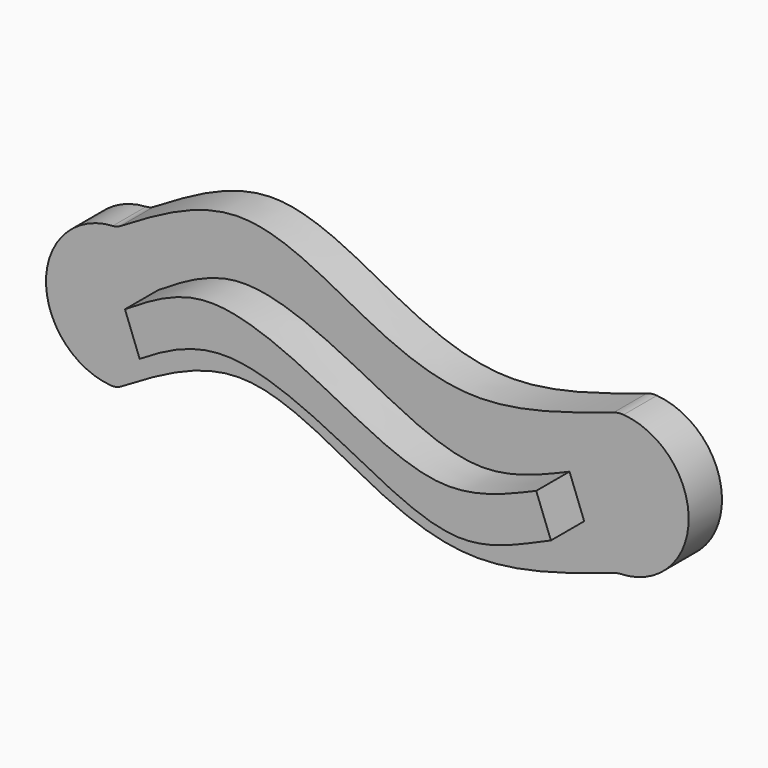
from build123d import *

# Parameters (mm, degrees)
F1_DEPTH = 12.7
F2_DEPTH = 25.4
F3_R     = 7.62
F4_R     = 5.08
F5_R     = 5.08
F6_R     = 5.08


# Not quite as in the source:
# - the program builds the solid bodies; features that only make, move or delete a surface that nothing else refers to are left out


with BuildPart() as f1:
    # F0 (on Front) → F1 (new body)
    with BuildSketch(Plane.XZ):
        with BuildLine():
            add(Edge.make_bspline(
                [(-76.5334740281, 20.7332828829), (-63.8515293548, 28.3869740492), (-38.487641079, 43.6943557355), (-0.1074870643, 19.2987869132), (33.6920782855, 6.372177087), (61.7287419774, 15.7705051868), (76.5334740281, 20.7332828829)],
                knots=[0, 0, 0, 0, 0.252598913, 0.5051978047, 0.7387201987, 1, 1, 1, 1], degree=3))
            Line((-76.5334740281, 20.7332828829), (-76.5334740281, -22.4467171171))
            add(Edge.make_bspline(
                [(-76.5334740281, -22.4467171171), (-63.8515293548, -14.7930259508), (-38.487641079, 0.5143557355), (-0.1074870643, -23.8812130868), (33.6920782855, -36.807822913), (61.7287419774, -27.4094948132), (76.5334740281, -22.4467171171)],
                knots=[0, 0, 0, 0, 0.252598913, 0.5051978047, 0.7387201987, 1, 1, 1, 1], degree=3))
            Line((76.5334740281, -22.4467171171), (76.5334740281, 20.7332828829))
        make_face()
        with BuildLine():
            Line((-59.3705394858, -3.9110629208), (-63.8515293548, 7.9721491784))
            add(Edge.make_bspline(
                [(-63.8515293548, 7.9721491784), (-55.8466582979, 13.0095149676), (-38.1452218943, 24.1488087208), (0.3419863459, 5.213337181), (32.9615149645, -12.272359942), (52.4893434663, -3.9416111996), (61.7287419774, 0)],
                knots=[0, 0, 0, 0, 0.228361581, 0.5049835251, 0.7657878611, 1, 1, 1, 1], degree=3))
            Line((61.7287419774, 0), (66.2097318464, -11.8832120992))
            add(Edge.make_bspline(
                [(-59.3705394858, -3.9110629208), (-51.3634228426, 1.1277159879), (-33.1115500983, 10.7952182475), (5.0660805533, -7.2965458084), (37.9471343056, -25.5812525078), (56.9802173789, -15.8206066761), (66.2097318464, -11.8832120992)],
                knots=[0, 0, 0, 0, 0.2284256427, 0.505143577, 0.7660384145, 1, 1, 1, 1], degree=3))
        make_face(mode=Mode.SUBTRACT)
        with BuildLine():
            Line((-76.5334740281, -22.4467171171), (-76.5334740281, 20.7332828829))
            ThreePointArc((-76.5334740281, 20.7332828829), (-98.1234740281, -0.8567171171), (-76.5334740281, -22.4467171171))
        make_face()
        with BuildLine():
            ThreePointArc((76.5334740281, -22.4467171171), (98.1234740281, -0.8567171171), (76.5334740281, 20.7332828829))
            Line((76.5334740281, 20.7332828829), (76.5334740281, -22.4467171171))
        make_face()
    extrude(amount=F1_DEPTH)

    # F0 (on Front) → F2 (join)
    with BuildSketch(Plane.XZ):
        with BuildLine():
            add(Edge.make_bspline(
                [(-63.8515293548, 7.9721491784), (-55.8466582979, 13.0095149676), (-38.1452218943, 24.1488087208), (0.3419863459, 5.213337181), (32.9615149645, -12.272359942), (52.4893434663, -3.9416111996), (61.7287419774, 0)],
                knots=[0, 0, 0, 0, 0.228361581, 0.5049835251, 0.7657878611, 1, 1, 1, 1], degree=3))
            Line((-63.8515293548, 7.9721491784), (-59.3705394858, -3.9110629208))
            add(Edge.make_bspline(
                [(-59.3705394858, -3.9110629208), (-51.3634228426, 1.1277159879), (-33.1115500983, 10.7952182475), (5.0660805533, -7.2965458084), (37.9471343056, -25.5812525078), (56.9802173789, -15.8206066761), (66.2097318464, -11.8832120992)],
                knots=[0, 0, 0, 0, 0.2284256427, 0.505143577, 0.7660384145, 1, 1, 1, 1], degree=3))
            Line((66.2097318464, -11.8832120992), (61.7287419774, 0))
        make_face()
    extrude(amount=F2_DEPTH)

    # F3
    f3_edges = [f1.edges().sort_by_distance(p)[0] for p in [
        (76.533474, -6.35, 20.733283),
    ]]
    fillet(f3_edges, radius=F3_R)

    # F4
    f4_edges = [f1.edges().sort_by_distance(p)[0] for p in [
        (-76.533474, -6.35, -22.446717),
    ]]
    fillet(f4_edges, radius=F4_R)

    # F5
    f5_edges = [f1.edges().sort_by_distance(p)[0] for p in [
        (-76.533474, -6.35, 20.733283),
    ]]
    fillet(f5_edges, radius=F5_R)

    # F6
    f6_edges = [f1.edges().sort_by_distance(p)[0] for p in [
        (76.533474, -6.35, -22.446717),
    ]]
    fillet(f6_edges, radius=F6_R)


solid = f1.part
